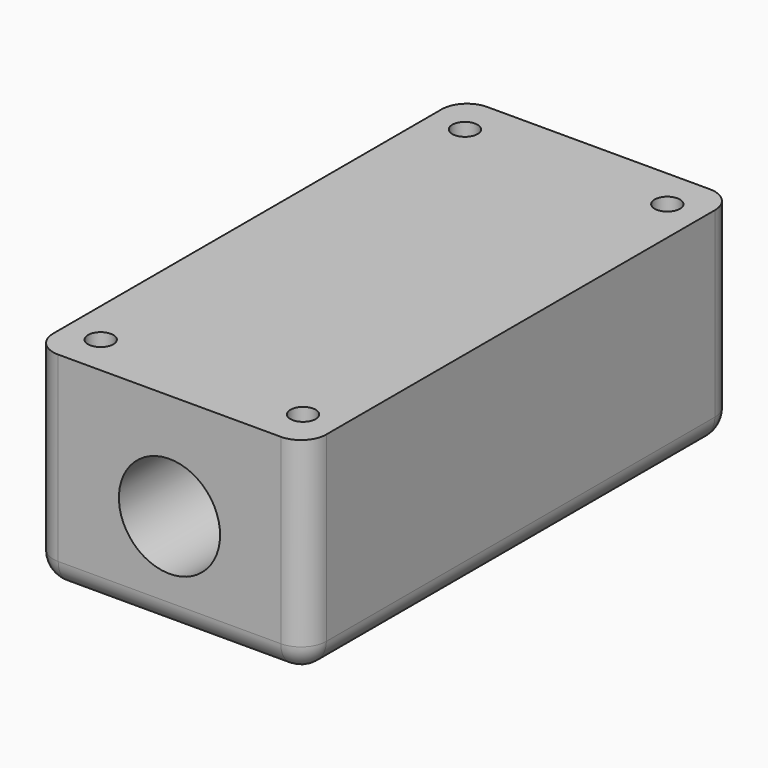
from build123d import *

# Parameters (mm, degrees)
F0_W         = 54
F0_H         = 41
F0_R         = 10
F1_DEPTH     = 106
F3_D         = 5
F4_T1_DEPTH  = 48.5
F4_T3_DEPTH  = 44
F4_T5_DEPTH  = 96
F4_S9_W      = 5
F4_S9_H      = 5
F4_T10_DEPTH = 5
F4_S15_W     = 5
F4_S15_H     = 5
F4_T16_DEPTH = 5
F4_S21_W     = 5
F4_S21_H     = 5
F4_T22_DEPTH = 5
F4_S27_W     = 5
F4_S27_H     = 5
F4_T28_DEPTH = 5


# Not quite as in the source:
# - a fillet or chamfer that OpenCascade refuses, or shapes differently, is made with other operations: its cross-section is extruded or revolved along the edge and cut away or added


with BuildPart() as f1:
    # F0 (on Front) → F1 (new body)
    with BuildSketch(Plane.XZ):
        Rectangle(F0_W, F0_H)
        with Locations((0, -0.5)):
            Circle(F0_R, mode=Mode.SUBTRACT)
    extrude(amount=F1_DEPTH)

    # F3 (through all)
    with Locations(Plane.XY.offset(20.5)):
        with Locations((-20, -8), (20, -8), (-20, -98), (20, -98)):
            Hole(F3_D / 2)

    # F4: fillet of radius 5 on 8 edges, made by hand

    # F4_s2 → F4_t1 (cut)
    with BuildSketch(Plane.XY.offset(-15.5)):
        with BuildLine():
            ThreePointArc((-22, -106), (-25.5355339059, -104.5355339059), (-27, -101))
            Line((-27, -101), (-27, -106))
            Line((-27, -106), (-22, -106))
        make_face()
        with BuildLine():
            ThreePointArc((27, -101), (25.5355339059, -104.5355339059), (22, -106))
            Line((22, -106), (27, -106))
            Line((27, -106), (27, -101))
        make_face()
        with BuildLine():
            ThreePointArc((27, -5), (25.5355339059, -1.4644660941), (22, 0))
            Line((22, 0), (27, 0))
            Line((27, 0), (27, -5))
        make_face()
        with BuildLine():
            ThreePointArc((-22, 0), (-25.5355339059, -1.4644660941), (-27, -5))
            Line((-27, -5), (-27, 0))
            Line((-27, 0), (-22, 0))
        make_face()
    extrude(amount=F4_T1_DEPTH, mode=Mode.SUBTRACT)

    # F4_s4 → F4_t3 (cut)
    with BuildSketch(Plane.YZ.offset(-22)):
        with BuildLine():
            ThreePointArc((-101, -20.5), (-104.5355339059, -19.0355339059), (-106, -15.5))
            Line((-106, -15.5), (-106, -20.5))
            Line((-106, -20.5), (-101, -20.5))
        make_face()
        with BuildLine():
            ThreePointArc((-5, -20.5), (-1.4644660941, -19.0355339059), (0, -15.5))
            Line((0, -15.5), (0, -20.5))
            Line((0, -20.5), (-5, -20.5))
        make_face()
    extrude(amount=F4_T3_DEPTH, mode=Mode.SUBTRACT)

    # F4_s6 → F4_t5 (cut)
    with BuildSketch(Plane.XZ.offset(5)):
        with BuildLine():
            ThreePointArc((27, -15.5), (25.5355339059, -19.0355339059), (22, -20.5))
            Line((22, -20.5), (27, -20.5))
            Line((27, -20.5), (27, -15.5))
        make_face()
        with BuildLine():
            ThreePointArc((-22, -20.5), (-25.5355339059, -19.0355339059), (-27, -15.5))
            Line((-27, -15.5), (-27, -20.5))
            Line((-27, -20.5), (-22, -20.5))
        make_face()
    extrude(amount=F4_T5_DEPTH, mode=Mode.SUBTRACT)


with BuildPart() as f4_tool8:
    # F4_s9 → F4_t10 (new body)
    with BuildSketch(Plane.XY.offset(-15.5)):
        with Locations((-24.5, -103.5)):
            Rectangle(F4_S9_W, F4_S9_H)
    extrude(amount=-F4_T10_DEPTH)

    # F4_s11 → F4_t12 (revolve, cut)
    with BuildSketch(Plane(origin=(-22, -101, -15.5), x_dir=(0.7071067812, 0.7071067812, 0), z_dir=(-0.7071067812, 0.7071067812, 0))):
        with BuildLine():
            ThreePointArc((0, -5), (5, 0), (0, 5))
            Line((0, 5), (0, -5))
        make_face()
    revolve(axis=Axis((-22, -101, -15.5), (0, 0, -1)), mode=Mode.SUBTRACT)


with BuildPart() as f1_1:
    add(f1.part)

    # F4_t7: cut F4_tool8
    add(f4_tool8.part, mode=Mode.SUBTRACT)


with BuildPart() as f4_tool14:
    # F4_s15 → F4_t16 (new body)
    with BuildSketch(Plane.YZ.offset(22)):
        with Locations((-103.5, -18)):
            Rectangle(F4_S15_W, F4_S15_H)
    extrude(amount=F4_T16_DEPTH)

    # F4_s17 → F4_t18 (revolve, cut)
    with BuildSketch(Plane(origin=(22, -101, -15.5), x_dir=(0, 0.7071067812, 0.7071067812), z_dir=(0, 0.7071067812, -0.7071067812))):
        with BuildLine():
            ThreePointArc((0, -5), (5, 0), (0, 5))
            Line((0, 5), (0, -5))
        make_face()
    revolve(axis=Axis((22, -101, -15.5), (1, 0, 0)), mode=Mode.SUBTRACT)


with BuildPart() as f1_2:
    add(f1_1.part)

    # F4_t13: cut F4_tool14
    add(f4_tool14.part, mode=Mode.SUBTRACT)


with BuildPart() as f4_tool20:
    # F4_s21 → F4_t22 (new body)
    with BuildSketch(Plane.YZ.offset(22)):
        with Locations((-2.5, -18)):
            Rectangle(F4_S21_W, F4_S21_H)
    extrude(amount=F4_T22_DEPTH)

    # F4_s23 → F4_t24 (revolve, cut)
    with BuildSketch(Plane(origin=(22, -5, -15.5), x_dir=(0, -0.7071067812, 0.7071067812), z_dir=(0, 0.7071067812, 0.7071067812))):
        with BuildLine():
            ThreePointArc((0, -5), (5, 0), (0, 5))
            Line((0, 5), (0, -5))
        make_face()
    revolve(axis=Axis((22, -5, -15.5), (1, 0, 0)), mode=Mode.SUBTRACT)


with BuildPart() as f1_3:
    add(f1_2.part)

    # F4_t19: cut F4_tool20
    add(f4_tool20.part, mode=Mode.SUBTRACT)


with BuildPart() as f4_tool26:
    # F4_s27 → F4_t28 (new body)
    with BuildSketch(Plane.XY.offset(-15.5)):
        with Locations((-24.5, -2.5)):
            Rectangle(F4_S27_W, F4_S27_H)
    extrude(amount=-F4_T28_DEPTH)

    # F4_s29 → F4_t30 (revolve, cut)
    with BuildSketch(Plane(origin=(-22, -5, -15.5), x_dir=(0.7071067812, -0.7071067812, 0), z_dir=(0.7071067812, 0.7071067812, 0))):
        with BuildLine():
            ThreePointArc((0, -5), (5, 0), (0, 5))
            Line((0, 5), (0, -5))
        make_face()
    revolve(axis=Axis((-22, -5, -15.5), (0, 0, -1)), mode=Mode.SUBTRACT)


with BuildPart() as f1_4:
    add(f1_3.part)

    # F4_t25: cut F4_tool26
    add(f4_tool26.part, mode=Mode.SUBTRACT)


solid = f1_4.part
